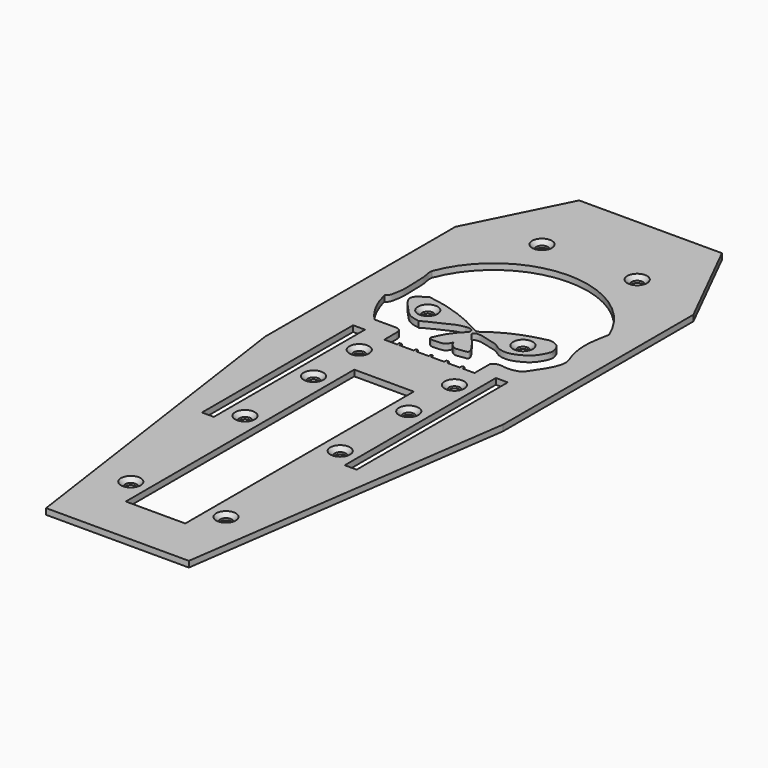
from build123d import *

# Parameters (mm, degrees)
F1_DEPTH       = 3.175
F3_DEPTH       = 3.176
F4_W           = 6.35
F4_H           = 100.8313270181
F4_W_2         = 31.75
F4_H_2         = 63.5
F4_H_3         = 25.4
F5_DEPTH       = 3.1760001
F7_D           = 6
F7_CSINK_D     = 10.5
F7_CSINK_ANGLE = 94


# Not quite as in the source:
# - a feature names something its author has since deleted; it is built from what else it names


with BuildPart() as f1:
    # F0 (on Top) → F1 (new body)
    with BuildSketch(Plane.XY):
        Polygon((38.1, -177.8), (63.5, 0), (63.5, 127), (38.1, 177.8), (-38.1, 177.8), (-63.5, 127), (-63.5, 0), (-38.1, -177.8), align=None)
    extrude(amount=F1_DEPTH)

    # F2 (on face) → F3 (cut, through all)
    with BuildSketch(Plane.XY.offset(3.175)):
        with BuildLine():
            add(Edge.make_bspline(
                [(25.1466520131, 39.4014343619), (25.6541484105, 39.9097199936), (26.7410176089, 40.9982794392), (29.802267098, 41.355245877), (32.692263509, 40.4595478573), (37.6570335333, 41.0972759164), (40.7302249381, 42.6825537331), (43.7038213764, 47.8612868255), (46.9401102159, 52.2202858755), (49.6208840062, 59.2330852617), (48.2033605352, 63.8134515414), (46.5104075294, 68.069113223), (45.8490539683, 72.6307041832), (45.4637153829, 76.3833853566), (45.6470407378, 80.9465541118), (46.1803556301, 84.3474374397), (46.8089873552, 88.077211433), (47.2151789569, 89.9454884702), (47.4034715641, 90.8115397446)],
                knots=[0, 0, 0, 0, 0.0455469265, 0.0975446362, 0.1520281706, 0.2196808725, 0.2765455384, 0.3498782935, 0.42422109, 0.5066378593, 0.5731201257, 0.6390538453, 0.7048593186, 0.7654118037, 0.8307237038, 0.8888652689, 0.9484828141, 1, 1, 1, 1], degree=3))
            ThreePointArc((47.4034715641, 90.8115397446), (0.2180060415, 122.2654322495), (-46.1966395378, 89.6848216653))
            add(Edge.make_bspline(
                [(-48.0537861586, 60.265570879), (-47.5034013978, 60.7457521416), (-46.3356042482, 61.764592687), (-45.7708233794, 64.5217799496), (-44.9436534796, 68.9541934356), (-45.1107622611, 73.3644028891), (-45.3932498796, 79.2957117589), (-45.350204679, 83.6167252081), (-46.4035424703, 87.3383295462), (-46.25972014, 88.9694227387), (-46.1966395378, 89.6848216653)],
                knots=[0, 0, 0, 0, 0.0957108325, 0.2030776383, 0.3406274201, 0.4798288902, 0.6381520421, 0.7757313325, 0.9016355627, 1, 1, 1, 1], degree=3))
            add(Edge.make_bspline(
                [(-48.0537861586, 60.265570879), (-45.9844991565, 52.1586798131), (-42.6741428673, 45.9517613053), (-37.5017113984, 40.5724346638)],
                knots=[0, 0, 0, 0, 22.3420208517, 22.3420208517, 22.3420208517, 22.3420208517], degree=3))
            Line((-37.5017113984, 40.5724346638), (-25.9372889996, 40.5724346638))
            ThreePointArc((-25.9372889996, 40.5724346638), (-23.8310435267, 39.6736239569), (-23.0226702988, 37.5310406089))
            Line((-23.0226702988, 37.5310406089), (-23.0226702988, 28.9468616247))
            Line((-23.0226702988, 28.9468616247), (-16.0195790231, 28.9468616247))
            add(Edge.make_bspline(
                [(-16.0195790231, 28.9468616247), (-16.0832569117, 29.1624848684), (-16.2122556873, 29.5992948043), (-16.2129852016, 30.5562231913), (-15.4025113931, 30.4769426012), (-14.4487840914, 30.5022395177), (-14.7284171354, 29.5622399817), (-14.820721123, 29.148947927), (-14.865854755, 28.9468616247)],
                knots=[0, 0, 0, 0, 0.1661668324, 0.3366210534, 0.4998235464, 0.6700995035, 0.8386894432, 1, 1, 1, 1], degree=3))
            Line((-14.865854755, 28.9468616247), (-7.2567402385, 28.9468616247))
            add(Edge.make_bspline(
                [(-7.2567402385, 28.9468616247), (-7.3110800528, 29.1863895794), (-7.415097758, 29.6448958984), (-7.2577090782, 30.2531850516), (-6.8120795253, 30.6584082243), (-6.047603364, 30.4118052636), (-5.8927532747, 29.6904809929), (-5.9961810993, 29.2006761887), (-6.0497769155, 28.9468616247)],
                knots=[0, 0, 0, 0, 0.1744634922, 0.3339594066, 0.4833295227, 0.6513235418, 0.8193174863, 1, 1, 1, 1], degree=3))
            Line((-6.0497769155, 28.9468616247), (0.6813724758, 28.9468616247))
            add(Edge.make_bspline(
                [(0.6813724758, 28.9468616247), (0.6612179066, 29.0618807965), (0.6148402246, 29.3265514296), (0.5758060371, 29.9803746589), (0.9947753255, 30.5705129645), (1.7504166408, 30.4936355843), (1.9146407509, 30.0082897467), (1.9942363671, 29.619356366), (1.901134685, 29.1909107695), (1.8481025472, 28.9468616247)],
                knots=[0, 0, 0, 0, 0.1197669688, 0.2755957893, 0.4322060703, 0.5858081726, 0.7162215613, 0.8383554742, 1, 1, 1, 1], degree=3))
            Line((1.8481025472, 28.9468616247), (8.905894123, 28.9468616247))
            add(Edge.make_bspline(
                [(8.905894123, 28.9468616247), (8.8968815712, 29.0869069656), (8.8776848364, 29.385203532), (8.8175679877, 29.9580165392), (9.0998757779, 30.4458940104), (9.9238543438, 30.5058467732), (10.3695051194, 30.4092160475), (10.8853542049, 29.9366290742), (10.7091636532, 29.4691389939), (10.5908009754, 29.1279369659), (10.5279861018, 28.9468616247)],
                knots=[0, 0, 0, 0, 0.1129855079, 0.2406591238, 0.3603192713, 0.5087573063, 0.6273257155, 0.7588596696, 0.8720272331, 1, 1, 1, 1], degree=3))
            Line((10.5279861018, 28.9468616247), (17.2053873539, 28.9468616247))
            add(Edge.make_bspline(
                [(17.2053873539, 28.9468616247), (17.2244810946, 29.0925659518), (17.2655541771, 29.4059946252), (17.1521143713, 30.0690005026), (17.4840461934, 30.3527026136), (17.8613601128, 30.6539121174), (18.4491638149, 30.6363427059), (18.8631597524, 30.3909043183), (18.9901386523, 29.7860292038), (18.7710317888, 29.2858556713), (18.7947431142, 29.0500438164), (18.8051182777, 28.9468616247)],
                knots=[0, 0, 0, 0, 0.1097112007, 0.2360028476, 0.336333599, 0.4458711072, 0.5648198983, 0.6712927079, 0.7916835706, 0.9088487482, 1, 1, 1, 1], degree=3))
            Line((18.8051182777, 28.9468616247), (25.1466520131, 28.9468616247))
            Line((25.1466520131, 28.9468616247), (25.1466520131, 39.4014343619))
        make_face()
        with BuildLine():
            add(Edge.make_bspline(
                [(-32.5099825859, 70.8164721727), (-33.4767643979, 70.0386899104), (-35.1551652981, 68.6883877902), (-36.8788013086, 67.794350095), (-38.5240687275, 65.5337143611), (-37.6296964893, 62.6061764402), (-34.383372811, 58.772552848), (-31.4645623193, 55.4949813977), (-28.0103280735, 52.1546915998), (-24.425201544, 51.3989492118), (-22.3055128008, 51.0394908488)],
                knots=[0, 0, 0, 0, 0.1201835941, 0.2109499126, 0.3124503406, 0.4210186762, 0.5665973859, 0.7048496115, 0.8433597144, 1, 1, 1, 1], degree=3))
            add(Edge.make_bspline(
                [(-32.5099825859, 70.8164721727), (-19.7686786141, 69.1300872499), (-9.0976193008, 64.9904033457), (0.5971823463, 59.4714263061)],
                knots=[0, 0, 0, 0, 34.8655276916, 34.8655276916, 34.8655276916, 34.8655276916], degree=3))
            add(Edge.make_bspline(
                [(0.5971823463, 59.4714263061), (0.7820097594, 59.3662092748), (0.9664823432, 59.2604909275), (1.1506076782, 59.1542787064)],
                knots=[34.8655276916, 34.8655276916, 34.8655276916, 34.8655276916, 35.5302246623, 35.5302246623, 35.5302246623, 35.5302246623], degree=3))
            add(Edge.make_bspline(
                [(1.1506076782, 59.1542787064), (2.1026312697, 58.7087277222), (2.9564514091, 58.832758493), (3.6766339037, 59.3454347331)],
                knots=[0.4866340364, 0.4866340364, 0.4866340364, 0.4866340364, 3.0461411723, 3.0461411723, 3.0461411723, 3.0461411723], degree=3))
            add(Edge.make_bspline(
                [(3.8414998047, 59.4714263061), (3.7864188033, 59.429500042), (3.7314614526, 59.3875020213), (3.6766339037, 59.3454347331)],
                knots=[0.8631102569, 0.8631102569, 0.8631102569, 0.8631102569, 0.8642336328, 0.8642336328, 0.8642336328, 0.8642336328], degree=3))
            add(Edge.make_bspline(
                [(1.1248061201, 45.0130552053), (1.2833485432, 44.5669486437), (1.6225154831, 43.6126192798), (2.8978459963, 42.1865316915), (4.6349767377, 41.1322648961), (6.758990357, 41.3152946659), (10.1045617952, 41.8043543653), (11.4305546663, 42.096437936), (11.2583594734, 43.9161109754), (9.2782782143, 46.9085165665), (7.4965961168, 49.3455069349), (5.6254821843, 51.4509041808), (3.4065512728, 54.3013152549), (2.06502352, 55.6217977372), (2.4893249595, 57.0133307749), (4.6105512863, 57.3973754433), (7.5161284834, 56.9810141568), (11.8387250438, 55.8573247428), (16.4299371669, 54.7147429842), (19.0120753503, 52.1768197136), (23.0719371266, 51.5276565125), (26.2524019007, 51.811770589), (30.3216873354, 53.5665423205), (33.7854623784, 55.7290373148), (36.3647776928, 58.9132973073), (38.838039743, 63.7894991526), (38.1033822684, 66.4588968174), (37.1117810977, 69.1950497663), (34.8280376409, 70.8895851689), (31.4076096004, 71.5858034404), (30.6751906198, 71.2657910318), (25.0851818192, 70.0152733481), (20.3209789449, 68.535586985), (13.8020483064, 65.8318889547), (8.6325614613, 62.8730330148), (5.2380313326, 60.5344307578), (3.8414998047, 59.4714263061)],
                knots=[0, 0, 0, 0, 0.017320636, 0.037055297, 0.0568568123, 0.077990518, 0.1046702542, 0.1196140486, 0.1367176793, 0.164181802, 0.1893609715, 0.2136505214, 0.2411572842, 0.2600637705, 0.2748045019, 0.2946041462, 0.319369055, 0.3500357539, 0.3810805972, 0.4079754393, 0.4362077016, 0.4619721996, 0.4919073561, 0.5207382018, 0.5501563547, 0.582959266, 0.606324531, 0.6300485149, 0.6545298592, 0.6802347006, 0.6933153817, 0.7262935085, 0.7600211712, 0.7976071381, 0.8346280235, 0.8631102569, 0.8631102569, 0.8631102569, 0.8631102569], degree=3))
            add(Edge.make_bspline(
                [(-9.16706305, 42.4386039376), (-9.0714448048, 42.2439695099), (-8.8879495098, 41.7785763899), (-7.7021443285, 41.2023643401), (-6.5271635777, 41.1165197803), (-4.2175888812, 41.2568745964), (-2.3001918077, 41.4026721893), (-0.3907671548, 41.9445713168), (0.562225675, 43.9241573744), (0.9545689823, 44.6833856908), (1.1248061201, 45.0130552053)],
                knots=[0, 0, 0, 0, 0.0834881865, 0.1949521068, 0.3069464418, 0.4600524039, 0.6036003804, 0.7415325449, 0.8878610734, 1, 1, 1, 1], degree=3))
            add(Edge.make_bspline(
                [(0, 56.2095832163), (-0.7464119613, 55.4963225975), (-2.8599015538, 53.3146689644), (-5.8199409898, 49.4755753155), (-7.7759022948, 45.5869001502), (-8.7228545792, 43.4438794539), (-9.16706305, 42.4386039376)],
                knots=[0.891200272, 0.891200272, 0.891200272, 0.891200272, 0.9089129474, 0.9437824389, 0.9736301868, 1, 1, 1, 1], degree=3))
            add(Edge.make_bspline(
                [(-3.6333180033, 59.1700784862), (0, 59.6856512129), (0.9321252583, 57.6008036733), (0, 56.2095832163)],
                knots=[0, 0, 0, 0, 4.6867400137, 4.6867400137, 4.6867400137, 4.6867400137], degree=3))
            add(Edge.make_bspline(
                [(-22.3055128008, 51.0394908488), (-21.2718414205, 51.7745252194), (-18.8666358706, 52.9881029477), (-16.433967029, 54.224272636), (-11.5350652759, 56.5533929316), (-7.8398691568, 58.3000111791), (-5.0801757104, 58.8873815806), (-3.6333180033, 59.1700784862)],
                knots=[0, 0, 0, 0, 0.1952178046, 0.3630543934, 0.5917363756, 0.7955952722, 1, 1, 1, 1], degree=3))
        make_face(mode=Mode.SUBTRACT)
        with BuildLine():
            add(Edge.make_bspline(
                [(0.5971823463, 59.4714263061), (0.7820097594, 59.3662092748), (0.9664823432, 59.2604909275), (1.1506076782, 59.1542787064)],
                knots=[34.8655276916, 34.8655276916, 34.8655276916, 34.8655276916, 35.5302246623, 35.5302246623, 35.5302246623, 35.5302246623], degree=3))
            add(Edge.make_bspline(
                [(0.5971823463, 59.4714263061), (0.7850450242, 59.3442917841), (0.9696013131, 59.238990435), (1.1506076782, 59.1542787064)],
                knots=[0, 0, 0, 0, 0.4866340364, 0.4866340364, 0.4866340364, 0.4866340364], degree=3))
        make_face()
        with BuildLine():
            add(Edge.make_bspline(
                [(3.8414998047, 59.4714263061), (3.7864188033, 59.429500042), (3.7314614526, 59.3875020213), (3.6766339037, 59.3454347331)],
                knots=[0.8631102569, 0.8631102569, 0.8631102569, 0.8631102569, 0.8642336328, 0.8642336328, 0.8642336328, 0.8642336328], degree=3))
            add(Edge.make_bspline(
                [(3.6766339037, 59.3454347331), (3.7323958471, 59.3851299821), (3.78735663, 59.4271551688), (3.8414998047, 59.4714263061)],
                knots=[3.0461411723, 3.0461411723, 3.0461411723, 3.0461411723, 3.2443174584, 3.2443174584, 3.2443174584, 3.2443174584], degree=3))
        make_face()
    extrude(amount=-F3_DEPTH, mode=Mode.SUBTRACT)

    # F4 (on face) → F5 (cut, through all)
    with BuildSketch(Plane.XY.offset(3.175)):
        with Locations((-38.1, -19.4343364909)):
            Rectangle(F4_W, F4_H)
        with Locations((0, -120.65)):
            Rectangle(F4_W_2, F4_H_2)
        with Locations((0, -76.2)):
            Rectangle(F4_W_2, F4_H_3)
        with Locations((0, -31.75)):
            Rectangle(F4_W_2, F4_H_2)
        with Locations((38.1, -19.4343364909)):
            Rectangle(F4_W, F4_H)
    extrude(amount=-F5_DEPTH, mode=Mode.SUBTRACT)

    # F7 (through all)
    with Locations(Plane.XY.offset(3.175)):
        with Locations((-25.4, 137.16), (25.4, 137.16), (-25.4, 60.96), (25.4, 60.96), (-25.4, 15.24), (25.4, 15.24), (25.4, -137.16), (-25.4, -137.16), (-25.4, -60.96), (25.4, -60.96), (-25.4, -15.24), (25.4, -15.24)):
            CounterSinkHole(F7_D / 2, F7_CSINK_D / 2, counter_sink_angle=F7_CSINK_ANGLE)


solid = f1.part
